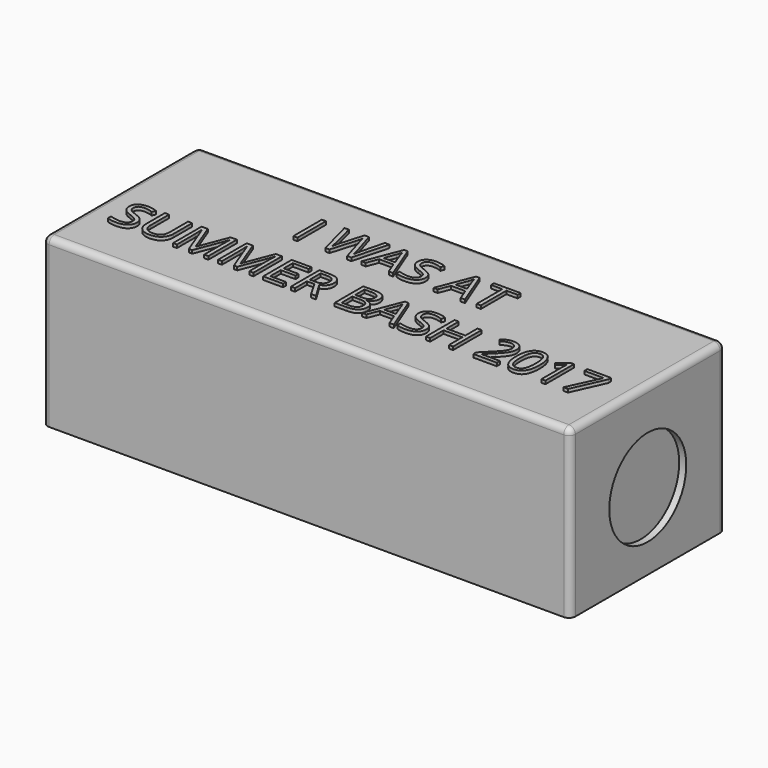
from build123d import *

# Parameters (mm, degrees)
F0_W         = 82.2
F0_H         = 30.2
F0_W_2       = 79.2
F0_H_2       = 27.2
F1_DEPTH     = 24
F3_START     = 24
F2_W         = 82.2
F2_H         = 30.2
F3_DEPTH     = 2
F4_R         = 1
F6_START     = 40
F5_R         = 6
F6_DEPTH     = 10
F7_START     = -40
F7_DEPTH     = 10
F8_TEXT_SIZE = 7.7761757416
F9_DEPTH     = 0.5
F11_START    = 40
F10_R        = 7.5
F11_DEPTH    = 10
F12_START    = -40
F12_DEPTH    = 10


# Not quite as in the source:
# - Text() gives the source's letters only with a copy of the font that has no kerning and outlines rounded to 1/6400 em; it was checked with that copy


with BuildPart() as f1:
    # F0 (on Top) → F1 (new body)
    with BuildSketch(Plane.XY):
        Rectangle(F0_W, F0_H)
        Rectangle(F0_W_2, F0_H_2, mode=Mode.SUBTRACT)
    extrude(amount=F1_DEPTH)

    # F2 (on Top) → F3 (join)
    with BuildSketch(Plane.XY.offset(F3_START)):
        Rectangle(F2_W, F2_H)
    extrude(amount=F3_DEPTH)

    # F4
    f4_edges = [f1.edges().sort_by_distance(p)[0] for p in [
        (-41.1, 0, 26),
        (0, -15.1, 26),
        (41.1, 0, 26),
        (0, 15.1, 26),
        (41.1, -15.1, 13),
        (-41.1, -15.1, 13),
        (41.1, 15.1, 13),
        (-41.1, 15.1, 13),
    ]]
    fillet(f4_edges, radius=F4_R)

    # F5 (on Front) → F6 (cut)
    with BuildSketch(Plane.XZ.offset(F6_START)):
        with Locations((0, 12)):
            Circle(F5_R)
    extrude(amount=F6_DEPTH, mode=Mode.SUBTRACT)

    # F5 (on Front) → F7 (cut)
    with BuildSketch(Plane.XZ.offset(F7_START)):
        with Locations((0, 12)):
            Circle(F5_R)
    extrude(amount=-F7_DEPTH, mode=Mode.SUBTRACT)

    # F8 (on face) → F9 (join)
    with BuildSketch(Plane.XY.offset(26)):
        with Locations((-17.2940933465, 3)):
            Text('I WAS AT', F8_TEXT_SIZE, font='Open Sans', text_align=(TextAlign.LEFT, TextAlign.BOTTOM))
        with Locations((-37.5, -7.5755990085)):
            Text('SUMMER BASH 2017', F8_TEXT_SIZE, font='Open Sans', text_align=(TextAlign.LEFT, TextAlign.BOTTOM))
    extrude(amount=F9_DEPTH)

    # F10 (on Right) → F11 (cut)
    with BuildSketch(Plane.YZ.offset(F11_START)):
        with Locations((0, 12)):
            Circle(F10_R)
    extrude(amount=F11_DEPTH, mode=Mode.SUBTRACT)

    # F10 (on Right) → F12 (cut)
    with BuildSketch(Plane.YZ.offset(F12_START)):
        with Locations((0, 12)):
            Circle(F10_R)
    extrude(amount=-F12_DEPTH, mode=Mode.SUBTRACT)


solid = f1.part
